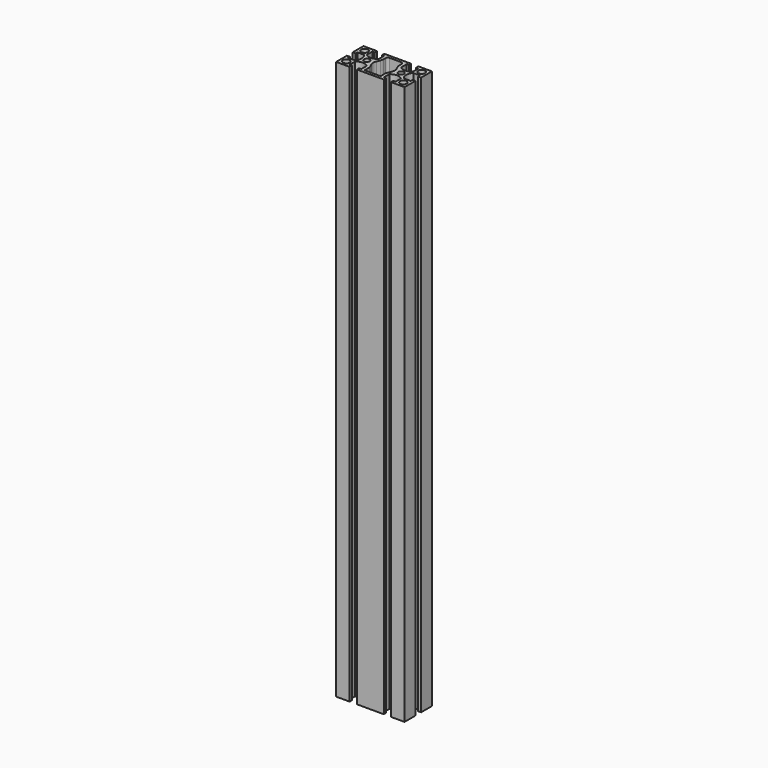
from build123d import *

# Parameters (mm, degrees)
F0_R     = 3
F0_R_2   = 2.5
F1_DEPTH = 490
F2_R     = 2
F3_R     = 7


# Not quite as in the source:
# - a feature names something its author has since deleted; it is built from what else it names


with BuildPart() as f1:
    # F0 (on Top) → F1 (new body)
    with BuildSketch(Plane.XY):
        with BuildLine():
            Line((18.15, -15), (30, -15))
            Line((30, -15), (30, -3.15))
            Line((30, -3.15), (27.5, -3.15))
            Line((27.5, -3.15), (27.5, -5.15))
            Line((27.5, -5.15), (21.5477069044, -5.15))
            ThreePointArc((21.5477069044, -5.15), (19.5, 0), (21.5477069044, 5.15))
            Line((21.5477069044, 5.15), (27.5, 5.15))
            Line((27.5, 5.15), (27.5, 3.15))
            Line((27.5, 3.15), (30, 3.15))
            Line((30, 3.15), (30, 15))
            Line((30, 15), (18.15, 15))
            Line((18.15, 15), (18.15, 12.5))
            Line((18.15, 12.5), (20.15, 12.5))
            Line((20.15, 12.5), (20.15, 6.5477069044))
            ThreePointArc((20.15, 6.5477069044), (15, 4.5), (9.85, 6.5477069044))
            Line((9.85, 6.5477069044), (9.85, 12.5))
            Line((9.85, 12.5), (11.85, 12.5))
            Line((11.85, 12.5), (11.85, 15))
            Line((11.85, 15), (-11.85, 15))
            Line((-11.85, 15), (-11.85, 12.5))
            Line((-11.85, 12.5), (-9.85, 12.5))
            Line((-9.85, 12.5), (-9.85, 6.5477069044))
            ThreePointArc((-9.85, 6.5477069044), (-15, 4.5), (-20.15, 6.5477069044))
            Line((-20.15, 6.5477069044), (-20.15, 12.5))
            Line((-20.15, 12.5), (-18.15, 12.5))
            Line((-18.15, 12.5), (-18.15, 15))
            Line((-18.15, 15), (-30, 15))
            Line((-30, 15), (-30, 3.15))
            Line((-30, 3.15), (-27.5, 3.15))
            Line((-27.5, 3.15), (-27.5, 5.15))
            Line((-27.5, 5.15), (-21.5477069044, 5.15))
            ThreePointArc((-21.5477069044, 5.15), (-19.5, 0), (-21.5477069044, -5.15))
            Line((-21.5477069044, -5.15), (-27.5, -5.15))
            Line((-27.5, -5.15), (-27.5, -3.15))
            Line((-27.5, -3.15), (-30, -3.15))
            Line((-30, -3.15), (-30, -15))
            Line((-30, -15), (-18.15, -15))
            Line((-18.15, -15), (-18.15, -12.5))
            Line((-18.15, -12.5), (-20.15, -12.5))
            Line((-20.15, -12.5), (-20.15, -6.5477069044))
            ThreePointArc((-20.15, -6.5477069044), (-15, -4.5), (-9.85, -6.5477069044))
            Line((-9.85, -6.5477069044), (-9.85, -12.5))
            Line((-9.85, -12.5), (-11.85, -12.5))
            Line((-11.85, -12.5), (-11.85, -15))
            Line((-11.85, -15), (11.85, -15))
            Line((11.85, -15), (11.85, -12.5))
            Line((11.85, -12.5), (9.85, -12.5))
            Line((9.85, -12.5), (9.85, -6.5477069044))
            ThreePointArc((9.85, -6.5477069044), (15, -4.5), (20.15, -6.5477069044))
            Line((20.15, -6.5477069044), (20.15, -12.5))
            Line((20.15, -12.5), (18.15, -12.5))
            Line((18.15, -12.5), (18.15, -15))
        make_face()
        with Locations((-25, -10)):
            Circle(F0_R, mode=Mode.SUBTRACT)
        with Locations((25, -10)):
            Circle(F0_R, mode=Mode.SUBTRACT)
        with Locations((-15, 0)):
            Circle(F0_R_2, mode=Mode.SUBTRACT)
        with Locations((-25, 10)):
            Circle(F0_R, mode=Mode.SUBTRACT)
        Polygon((-7, 7), (-7, 12.5), (0, 12.5), (7, 12.5), (7, 7), (10, 0), (7, -7), (7, -12.5), (0, -12.5), (-7, -12.5), (-7, -7), (-10, 0), align=None, mode=Mode.SUBTRACT)
        with Locations((15, 0)):
            Circle(F0_R_2, mode=Mode.SUBTRACT)
        with Locations((25, 10)):
            Circle(F0_R, mode=Mode.SUBTRACT)
    extrude(amount=F1_DEPTH)

    # F2
    f2_edges = [f1.edges().sort_by_distance(p)[0] for p in [
        (-7, 12.5, 245),
        (7, 12.5, 245),
    ]]
    fillet(f2_edges, radius=F2_R)

    # F3
    f3_edges = [f1.edges().sort_by_distance(p)[0] for p in [
        (-7, 7, 245),
        (-10, 0, 245),
        (7, 7, 245),
        (10, 0, 245),
    ]]
    fillet(f3_edges, radius=F3_R)


solid = f1.part
